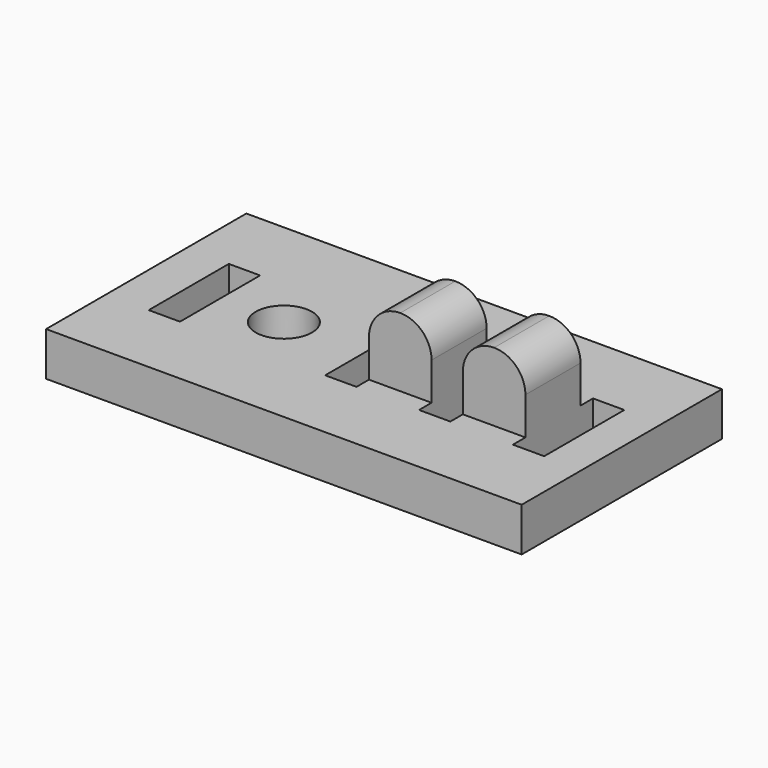
from build123d import *

# Parameters (mm, degrees)
F0_W     = 38
F0_H     = 20
F0_W_2   = 2.5
F0_H_2   = 8
F0_R     = 2.25
F1_DEPTH = 3.5
F2_W     = 5
F2_H     = 5.5
F3_DEPTH = 5.5
F4_R     = 2.49999


# Not quite as in the source:
# - a fillet or chamfer is up to 0.001 mm smaller than in the source, because OpenCascade refuses the exact size


with BuildPart() as f1:
    # F0 (on Top) → F1 (new body)
    with BuildSketch(Plane.XY):
        with Locations((11, -10)):
            Rectangle(F0_W, F0_H)
        with Locations((-3.3499999251, -10)):
            Rectangle(F0_W_2, F0_H_2, mode=Mode.SUBTRACT)
        with Locations((3, -10)):
            Circle(F0_R, mode=Mode.SUBTRACT)
        with Locations((10.75, -10)):
            Rectangle(F0_W_2, F0_H_2, mode=Mode.SUBTRACT)
        with Locations((18.25, -10)):
            Rectangle(F0_W_2, F0_H_2, mode=Mode.SUBTRACT)
        Polygon((24.5, -10), (24.5, -6), (27, -6), (27, -14), (24.5, -14), align=None, mode=Mode.SUBTRACT)
    extrude(amount=F1_DEPTH)

    # F2 (on face) → F3 (join)
    with BuildSketch(Plane.XY.offset(3.5)):
        with Locations((22, -10)):
            Rectangle(F2_W, F2_H)
        with Locations((14.5, -10)):
            Rectangle(F2_W, F2_H)
    extrude(amount=F3_DEPTH)

    # F4 (radius 2.5 in the source; OpenCascade refuses exactly that, so slightly less here)
    f4_edges = [f1.edges().sort_by_distance(p)[0] for p in [
        (12, -10, 9),
        (17, -10, 9),
        (19.5, -10, 9),
        (24.5, -10, 9),
    ]]
    fillet(f4_edges, radius=F4_R)


solid = f1.part
